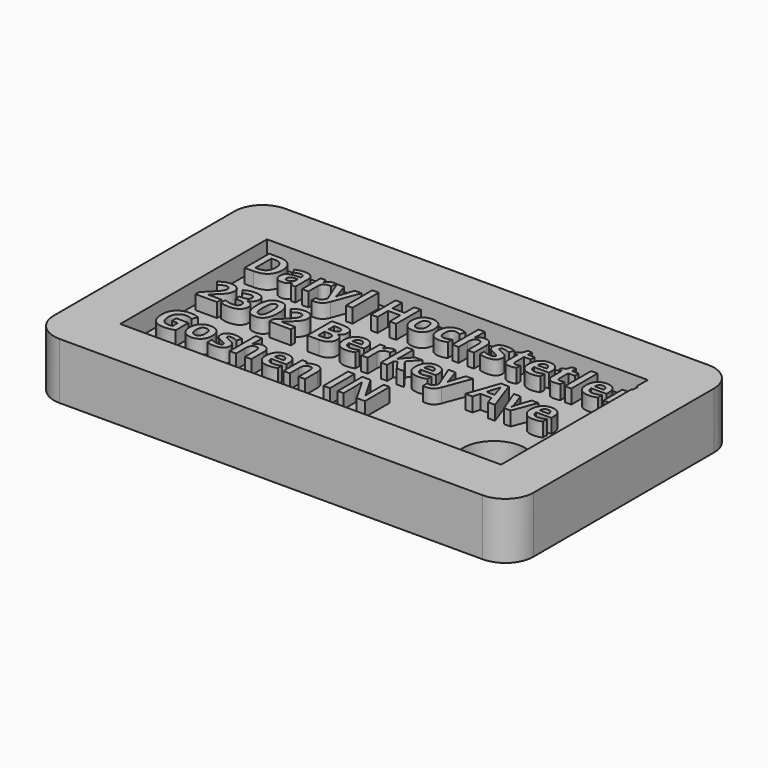
from build123d import *

# Parameters (mm, degrees)
F0_W         = 86.36
F0_H         = 50.8
F1_DEPTH     = 6.35
F2_TEXT_SIZE = 7.7611111111
F3_DEPTH     = 2.54
F4_R         = 5.588
F5_DEPTH     = 6.351
F6_W         = 86.36
F6_H         = 50.8
F7_DEPTH     = 3.81
F8_R         = 5.08


# Not quite as in the source:
# - Text() gives the source's letters only with a copy of the font that has no kerning and outlines rounded to 1/6400 em; it was checked with that copy


with BuildPart() as f1:
    # F0 (on Top) → F1 (new body)
    with BuildSketch(Plane.XY):
        Rectangle(F0_W, F0_H)
    extrude(amount=F1_DEPTH)

    # F2 (on face) → F3 (join)
    with BuildSketch(Plane.XY.offset(6.35)):
        with Locations((-33.528, 9.652)):
            Text('Daryl Hochstetler', F2_TEXT_SIZE, font='Open Sans', font_style=FontStyle.BOLD, text_align=(TextAlign.LEFT, TextAlign.BOTTOM))
        with Locations((-33.528, -0.9031111111)):
            Text('2302 Berkey Ave', F2_TEXT_SIZE, font='Open Sans', font_style=FontStyle.BOLD, text_align=(TextAlign.LEFT, TextAlign.BOTTOM))
        with Locations((-33.528, -11.4582222222)):
            Text('Goshen IN', F2_TEXT_SIZE, font='Open Sans', font_style=FontStyle.BOLD, text_align=(TextAlign.LEFT, TextAlign.BOTTOM))
    extrude(amount=F3_DEPTH)

    # F4 (on face) → F5 (cut, through all)
    with BuildSketch(Plane.XY.offset(6.35)):
        with Locations((27.94, -10.16)):
            Circle(F4_R)
    extrude(amount=-F5_DEPTH, mode=Mode.SUBTRACT)

    # F6 (on face) → F7 (join)
    with BuildSketch(Plane.XY.offset(6.35)):
        Rectangle(F6_W, F6_H)
        with BuildLine():
            Line((-34.29, -16.51), (-34.29, 16.51))
            Line((-34.29, 16.51), (34.29, 16.51))
            Line((34.29, 16.51), (34.29, 13.9655117935))
            add(Edge.make_bspline(
                [(34.5611979167, 13.9339505208), (34.4471880709, 13.9588901746), (34.29, 13.9655117935)],
                knots=[0, 0, 0, 0.7344943538, 0.7344943538, 0.7344943538], degree=2))
            Line((34.5611979167, 13.9339505208), (34.4738854167, 12.8510329861))
            add(Edge.make_bspline(
                [(34.29, 12.882059108), (34.3920081503, 12.8729139797), (34.4738854167, 12.8510329861)],
                knots=[2.1512313624, 2.1512313624, 2.1512313624, 2.3618421053, 2.3618421053, 2.3618421053], degree=2))
            Line((34.29, 12.882059108), (34.29, -16.51))
            Line((34.29, -16.51), (-34.29, -16.51))
        make_face(mode=Mode.SUBTRACT)
    extrude(amount=F7_DEPTH)

    # F8
    f8_edges = [f1.edges().sort_by_distance(p)[0] for p in [
        (-43.18, 25.4, 5.08),
        (-43.18, -25.4, 5.08),
        (43.18, 25.4, 5.08),
        (43.18, -25.4, 5.08),
    ]]
    fillet(f8_edges, radius=F8_R)


solid = f1.part
